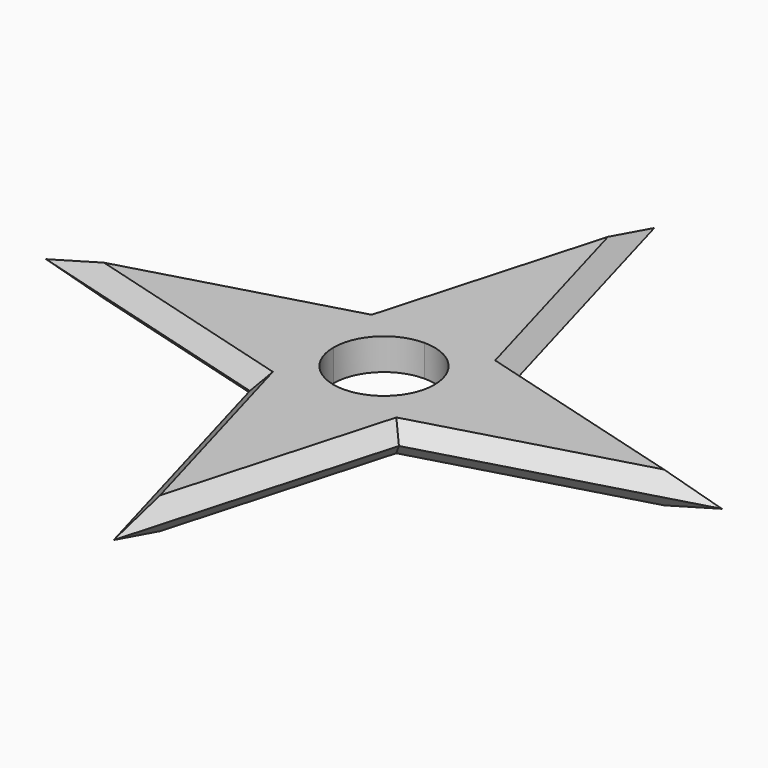
from build123d import *

# Parameters (mm, degrees)
F1_DEPTH = 7
F2_SIZE  = 3.5
F3_SIZE  = 3.49999


# Not quite as in the source:
# - a fillet or chamfer is up to 0.001 mm smaller than in the source, because OpenCascade refuses the exact size


with BuildPart() as f1:
    # F0 (on Top) → F1 (new body)
    with BuildSketch(Plane.XY):
        with BuildLine():
            ThreePointArc((-11.2, 0), (-7.9195959493, 7.9195959493), (0, 11.2))
            Line((0, 11.2), (0, 74.9999731779))
            Line((0, 74.9999731779), (-16.5413403588, 16.5413743234))
            Line((-16.5413403588, 16.5413743234), (-74.9999731779, 0))
            Line((-74.9999731779, 0), (-11.2, 0))
        make_face()
        with BuildLine():
            ThreePointArc((0, 11.2), (7.9195959493, 7.9195959493), (11.2, 0))
            Line((11.2, 0), (74.9999433756, 0))
            Line((74.9999433756, 0), (16.5414082881, 16.5413743234))
            Line((16.5414082881, 16.5413743234), (0, 74.9999731779))
            Line((0, 74.9999731779), (0, 11.2))
        make_face()
        with BuildLine():
            Line((74.9999433756, 0), (11.2, 0))
            ThreePointArc((11.2, 0), (7.9195959493, -7.9195959493), (0, -11.2))
            Line((0, -11.2), (0, -74.9999433756))
            Line((0, -74.9999433756), (16.5412724298, -16.5413063943))
            Line((16.5412724298, -16.5413063943), (74.9999433756, 0))
        make_face()
        with BuildLine():
            Line((0, -74.9999433756), (0, -11.2))
            ThreePointArc((0, -11.2), (-7.9195959493, -7.9195959493), (-11.2, 0))
            Line((-11.2, 0), (-74.9999731779, 0))
            Line((-74.9999731779, 0), (-16.5413403588, -16.5413063943))
            Line((-16.5413403588, -16.5413063943), (0, -74.9999433756))
        make_face()
    extrude(amount=F1_DEPTH)

    # F2
    f2_edges = [f1.edges().sort_by_distance(p)[0] for p in [
        (-45.770657, -8.270653, 7),
        (-8.27067, -45.770625, 7),
        (8.270636, -45.770625, 7),
        (45.770608, -8.270653, 7),
        (45.770676, 8.270687, 7),
        (8.270704, 45.770674, 7),
        (-8.27067, 45.770674, 7),
        (-45.770657, 8.270687, 7),
    ]]
    chamfer(f2_edges, length=F2_SIZE)

    # F3 (size 3.5 in the source; OpenCascade refuses exactly that, so slightly less here)
    f3_edges = [f1.edges().sort_by_distance(p)[0] for p in [
        (-45.770657, -8.270653, 0),
        (-45.770657, 8.270687, 0),
        (-8.27067, 45.770674, 0),
        (8.270704, 45.770674, 0),
        (45.770676, 8.270687, 0),
        (45.770608, -8.270653, 0),
        (8.270636, -45.770625, 0),
        (-8.27067, -45.770625, 0),
    ]]
    chamfer(f3_edges, length=F3_SIZE)


solid = f1.part
